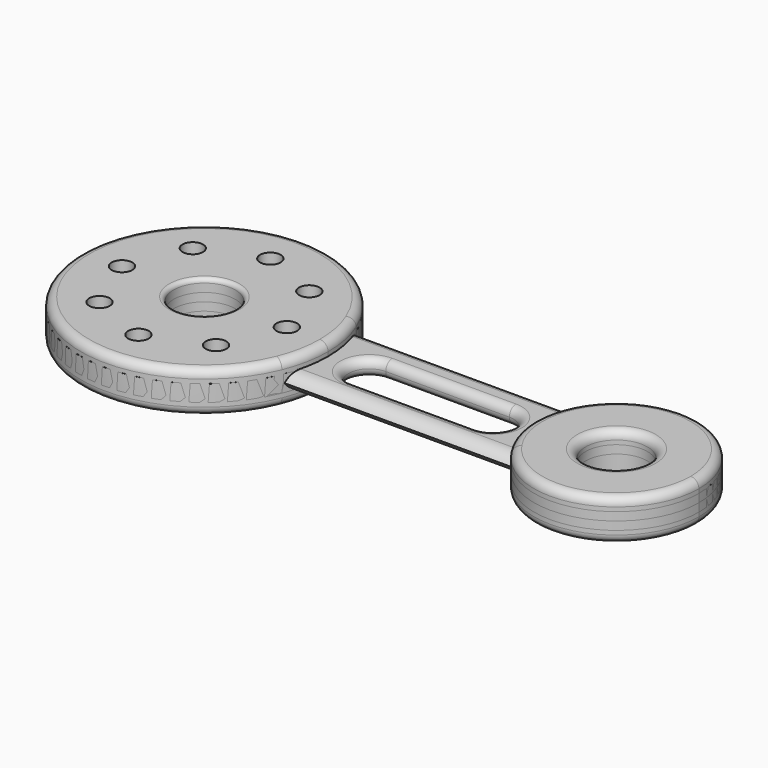
from build123d import *

# Parameters (mm, degrees)
F0_R         = 3.175
F0_R_2       = 9.525
F1_DEPTH     = 6.35
F2_DEPTH     = 2.54
F3_R         = 2.54
F3_2_R       = 2.54
F4_R         = 2.53999
F4_2_R       = 2.53999
F5_T4_DEPTH  = 96.0797036736
F5_S5_R      = 38.1
F5_T6_DEPTH  = 50
F5_S7_R      = 25.4
F5_T8_DEPTH  = 50
F5_T12_DEPTH = 96.0797036736
F5_S13_R     = 38.1
F5_T14_DEPTH = 50
F5_S15_R     = 25.4
F5_T16_DEPTH = 50
F6_R         = 1.27
F6_2_R       = 1.27


# Not quite as in the source:
# - a fillet or chamfer that OpenCascade refuses, or shapes differently, is made with other operations: its cross-section is extruded or revolved along the edge and cut away or added
# - a fillet or chamfer is up to 0.001 mm smaller than in the source, because OpenCascade refuses the exact size


with BuildPart() as f1:
    # F0 (on Top) → F1 (new body, symmetric)
    with BuildSketch(Plane.XY):
        with BuildLine():
            ThreePointArc((35.3196452948, -14.2875), (37.3984524127, -7.2777576996), (38.1, 0))
            ThreePointArc((38.1, 0), (37.3984524127, 7.2777576996), (35.3196452948, 14.2875))
            ThreePointArc((35.3196452948, 14.2875), (-38.1, 0), (35.3196452948, -14.2875))
        make_face()
        with Locations((0, -25.4)):
            Circle(F0_R, mode=Mode.SUBTRACT)
        with Locations((-17.9605122421, -17.9605122421)):
            Circle(F0_R, mode=Mode.SUBTRACT)
        with Locations((17.9605122421, -17.9605122421)):
            Circle(F0_R, mode=Mode.SUBTRACT)
        with Locations((-25.4, 0)):
            Circle(F0_R, mode=Mode.SUBTRACT)
        Circle(F0_R_2, mode=Mode.SUBTRACT)
        with Locations((-17.9605122421, 17.9605122421)):
            Circle(F0_R, mode=Mode.SUBTRACT)
        with Locations((25.4, 0)):
            Circle(F0_R, mode=Mode.SUBTRACT)
        with Locations((17.9605122421, 17.9605122421)):
            Circle(F0_R, mode=Mode.SUBTRACT)
        with Locations((0, 25.4)):
            Circle(F0_R, mode=Mode.SUBTRACT)
    extrude(amount=F1_DEPTH, both=True)

    # F3
    f3_edges = [f1.edges().sort_by_distance(p)[0] for p in [
        (-38.1, 0, 6.35),
        (-38.1, 0, -6.35),
    ]]
    fillet(f3_edges, radius=F3_R)

    # F6
    f6_edges = [f1.edges().sort_by_distance(p)[0] for p in [
        (-9.525, 0, 6.35),
        (-9.525, 0, -6.35),
    ]]
    fillet(f6_edges, radius=F6_R)


with BuildPart() as f1b:
    # F0 (on Top) → F1, piece 2 (new body, symmetric)
    with BuildSketch(Plane.XY):
        with BuildLine():
            ThreePointArc((152.4, 0), (134.4747395874, 24.2752604126), (105.9993489684, 14.2875))
            ThreePointArc((105.9993489684, 14.2875), (101.6, 0), (105.9993489684, -14.2875))
            ThreePointArc((105.9993489684, -14.2875), (134.4747395874, -24.2752604126), (152.4, 0))
        make_face()
        with Locations((127, 0)):
            Circle(F0_R_2, mode=Mode.SUBTRACT)
    extrude(amount=F1_DEPTH, both=True)

    # F3#2
    f3_2_edges = [f1b.edges().sort_by_distance(p)[0] for p in [
        (101.6, 0, 6.35),
        (101.6, 0, -6.35),
    ]]
    fillet(f3_2_edges, radius=F3_2_R)

    # F4#2 (radius 2.54 in the source; OpenCascade refuses exactly that, so slightly less here)
    f4_2_edges = [f1b.edges().sort_by_distance(p)[0] for p in [
        (117.475, 0, 6.35),
    ]]
    fillet(f4_2_edges, radius=F4_2_R)

    # F6#2
    f6_2_edges = [f1b.edges().sort_by_distance(p)[0] for p in [
        (117.475, 0, -6.35),
    ]]
    fillet(f6_2_edges, radius=F6_2_R)


with BuildPart() as f2:
    # F0 (on Top) → F2 (new body, symmetric)
    with BuildSketch(Plane.XY):
        with BuildLine():
            ThreePointArc((35.3196452948, -14.2875), (37.3984524127, -7.2777576996), (38.1, 0))
            ThreePointArc((38.1, 0), (37.3984524127, 7.2777576996), (35.3196452948, 14.2875))
            ThreePointArc((35.3196452948, 14.2875), (-38.1, 0), (35.3196452948, -14.2875))
        make_face()
        with Locations((0, -25.4)):
            Circle(F0_R, mode=Mode.SUBTRACT)
        with Locations((-17.9605122421, -17.9605122421)):
            Circle(F0_R, mode=Mode.SUBTRACT)
        with Locations((17.9605122421, -17.9605122421)):
            Circle(F0_R, mode=Mode.SUBTRACT)
        with Locations((-25.4, 0)):
            Circle(F0_R, mode=Mode.SUBTRACT)
        Circle(F0_R_2, mode=Mode.SUBTRACT)
        with Locations((-17.9605122421, 17.9605122421)):
            Circle(F0_R, mode=Mode.SUBTRACT)
        with Locations((25.4, 0)):
            Circle(F0_R, mode=Mode.SUBTRACT)
        with Locations((17.9605122421, 17.9605122421)):
            Circle(F0_R, mode=Mode.SUBTRACT)
        with Locations((0, 25.4)):
            Circle(F0_R, mode=Mode.SUBTRACT)
        with BuildLine():
            ThreePointArc((35.3196452948, 14.2875), (37.3984524127, 7.2777576996), (38.1, 0))
            ThreePointArc((38.1, 0), (37.3984524127, -7.2777576996), (35.3196452948, -14.2875))
            Line((35.3196452948, -14.2875), (105.9993489684, -14.2875))
            ThreePointArc((105.9993489684, -14.2875), (101.6, 0), (105.9993489684, 14.2875))
            Line((105.9993489684, 14.2875), (35.3196452948, 14.2875))
        make_face()
        with BuildLine():
            Line((88.9, -6.35), (50.8, -6.35))
            ThreePointArc((50.8, -6.35), (44.45, 0), (50.8, 6.35))
            Line((50.8, 6.35), (88.9, 6.35))
            ThreePointArc((88.9, 6.35), (95.25, 0), (88.9, -6.35))
        make_face(mode=Mode.SUBTRACT)
        with BuildLine():
            ThreePointArc((152.4, 0), (134.4747395874, 24.2752604126), (105.9993489684, 14.2875))
            ThreePointArc((105.9993489684, 14.2875), (101.6, 0), (105.9993489684, -14.2875))
            ThreePointArc((105.9993489684, -14.2875), (134.4747395874, -24.2752604126), (152.4, 0))
        make_face()
        with Locations((127, 0)):
            Circle(F0_R_2, mode=Mode.SUBTRACT)
    extrude(amount=F2_DEPTH, both=True)

    # F4 (radius 2.54 in the source; OpenCascade refuses exactly that, so slightly less here)
    f4_edges = [f2.edges().sort_by_distance(p)[0] for p in [
        (70.659497, 14.2875, 2.54),
        (70.659497, 14.2875, -2.54),
        (69.85, 6.35, 2.54),
        (69.85, -6.35, 2.54),
        (117.475, 0, -2.54),
        (69.85, -6.35, -2.54),
    ]]
    fillet(f4_edges, radius=F4_R)

    # F5: fillet of radius 5.08 on 2 edges, made by hand


with BuildPart() as f5_tool2:
    # F5_s3 → F5_t4 (new body)
    with BuildSketch(Plane.YZ.offset(22.6196452948)):
        with BuildLine():
            ThreePointArc((-9.2075, 2.54), (-12.7996024484, 1.0521024484), (-14.2875, -2.54))
            Line((-14.2875, -2.54), (-14.2875, 2.54))
            Line((-14.2875, 2.54), (-9.2075, 2.54))
        make_face()
    extrude(amount=F5_T4_DEPTH)

    # F5_s5 → F5_t6 (cut, symmetric)
    with BuildSketch(Plane.XY):
        Circle(F5_S5_R)
    extrude(amount=F5_T6_DEPTH, both=True, mode=Mode.SUBTRACT)

    # F5_s7 → F5_t8 (cut, symmetric)
    with BuildSketch(Plane.XY):
        with Locations((127, 0)):
            Circle(F5_S7_R)
    extrude(amount=F5_T8_DEPTH, both=True, mode=Mode.SUBTRACT)


with BuildPart() as f2_1:
    add(f2.part)

    # F5_t1: cut F5_tool2
    add(f5_tool2.part, mode=Mode.SUBTRACT)


with BuildPart() as f5_tool10:
    # F5_s11 → F5_t12 (new body)
    with BuildSketch(Plane.YZ.offset(22.6196452948)):
        with BuildLine():
            ThreePointArc((-9.2075, -2.54), (-12.7996024484, -1.0521024484), (-14.2875, 2.54))
            Line((-14.2875, 2.54), (-14.2875, -2.54))
            Line((-14.2875, -2.54), (-9.2075, -2.54))
        make_face()
    extrude(amount=F5_T12_DEPTH)

    # F5_s13 → F5_t14 (cut, symmetric)
    with BuildSketch(Plane.XY):
        Circle(F5_S13_R)
    extrude(amount=F5_T14_DEPTH, both=True, mode=Mode.SUBTRACT)

    # F5_s15 → F5_t16 (cut, symmetric)
    with BuildSketch(Plane.XY):
        with Locations((127, 0)):
            Circle(F5_S15_R)
    extrude(amount=F5_T16_DEPTH, both=True, mode=Mode.SUBTRACT)


with BuildPart() as f2_2:
    add(f2_1.part)

    # F5_t9: cut F5_tool10
    add(f5_tool10.part, mode=Mode.SUBTRACT)


solid = Compound([f1.part, f1b.part, f2_2.part])
